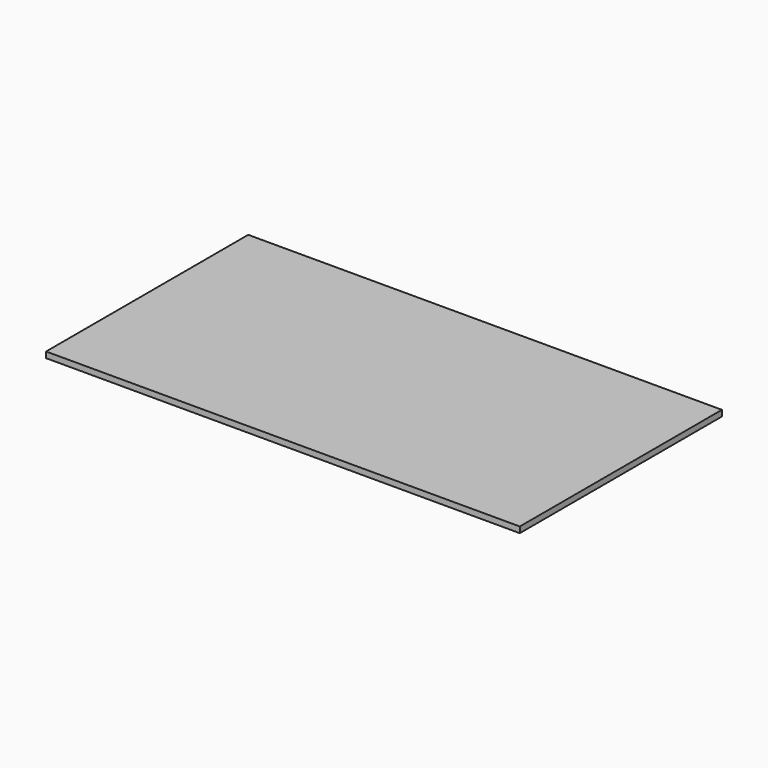
from build123d import *

# Parameters (mm, degrees)
F0_W     = 1524
F0_H     = 812.8
F0_W_2   = 1193.8
F0_H_2   = 609.6
F1_DEPTH = 19.05


# Not quite as in the source:
# - a feature names something its author has since deleted; it is built from what else it names


with BuildPart() as f1:
    # F0 (on Top) → F1 (new body)
    with BuildSketch(Plane.XY):
        Rectangle(F0_W, F0_H)
        with Locations((0, -50.8)):
            Rectangle(F0_W_2, F0_H_2, mode=Mode.SUBTRACT)
        with Locations((0, -50.8)):
            Rectangle(F0_W_2, F0_H_2)
    extrude(amount=-F1_DEPTH)


solid = f1.part
